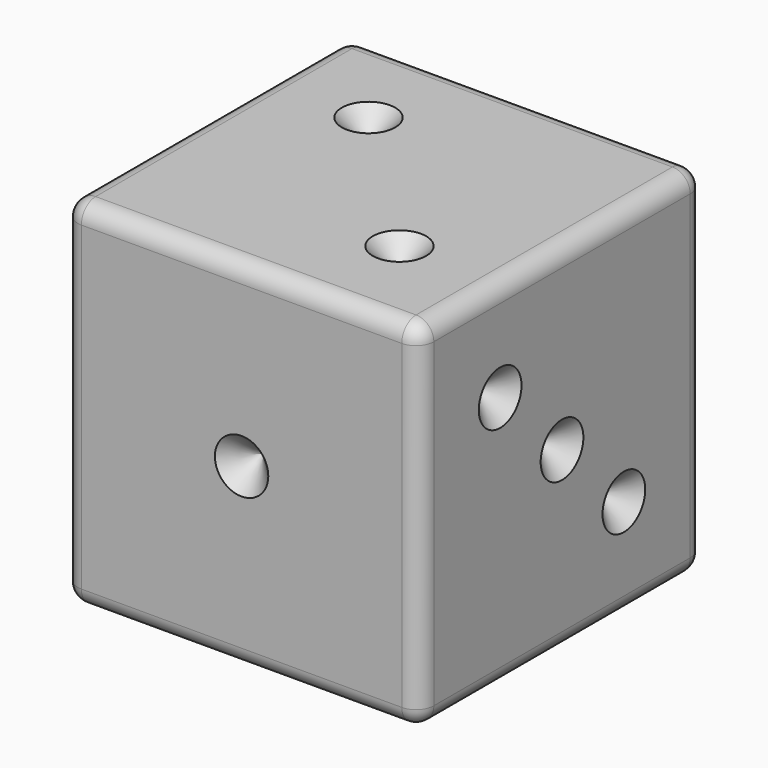
from build123d import *

# Parameters (mm, degrees)
F0_W      = 20
F0_H      = 20
F1_DEPTH  = 20
F2_R      = 1.5
F3_DEPTH  = 1.5
F4_R      = 1
F5_R      = 1.5
F6_DEPTH  = 1.5
F7_R      = 1.5
F8_DEPTH  = 1.5
F9_R      = 1.5
F10_DEPTH = 1.5
F11_R     = 1.5
F12_DEPTH = 1.5
F13_R     = 1.5
F14_DEPTH = 1.5
F15_SIZE  = 1.49999


# Not quite as in the source:
# - a fillet or chamfer is up to 0.001 mm smaller than in the source, because OpenCascade refuses the exact size


with BuildPart() as f1:
    # F0 (on Top) → F1 (new body)
    with BuildSketch(Plane.XY):
        with Locations((10, 10)):
            Rectangle(F0_W, F0_H)
    extrude(amount=F1_DEPTH)

    # F2 (on face) → F3 (cut)
    with BuildSketch(Plane.XZ):
        with Locations((10, 10)):
            Circle(F2_R)
    extrude(amount=-F3_DEPTH, mode=Mode.SUBTRACT)

    # F4
    f4_edges = [f1.edges().sort_by_distance(p)[0] for p in [
        (10, 0, 20),
        (20, 10, 20),
        (20, 0, 10),
        (0, 0, 10),
        (10, 0, 0),
        (20, 10, 0),
        (0, 10, 20),
        (10, 20, 20),
        (0, 10, 0),
        (0, 20, 10),
        (20, 20, 10),
        (10, 20, 0),
    ]]
    fillet(f4_edges, radius=F4_R)

    # F5 (on face) → F6 (cut)
    with BuildSketch(Plane.XY.offset(20)):
        with Locations((5.6568542495, 14.3431457505)):
            Circle(F5_R)
        with Locations((14.3431457505, 5.6568542495)):
            Circle(F5_R)
    extrude(amount=-F6_DEPTH, mode=Mode.SUBTRACT)

    # F7 (on face) → F8 (cut)
    with BuildSketch(Plane.YZ.offset(20)):
        with Locations((5.6568542495, 14.3431457505)):
            Circle(F7_R)
        with Locations((10, 10)):
            Circle(F7_R)
        with Locations((14.3431457505, 5.6568542495)):
            Circle(F7_R)
    extrude(amount=-F8_DEPTH, mode=Mode.SUBTRACT)

    # F9 (on face) → F10 (cut)
    with BuildSketch(Plane(origin=(0, 0, 0), x_dir=(0, -1, 0), z_dir=(-1, 0, 0))):
        with Locations((-14.3431457505, 14.3431457505)):
            Circle(F9_R)
        with Locations((-5.6568542495, 14.3431457505)):
            Circle(F9_R)
        with Locations((-14.3431457505, 5.6568542495)):
            Circle(F9_R)
        with Locations((-5.6568542495, 5.6568542495)):
            Circle(F9_R)
    extrude(amount=-F10_DEPTH, mode=Mode.SUBTRACT)

    # F11 (on face) → F12 (cut)
    with BuildSketch(Plane(origin=(0, 0, 0), x_dir=(1, 0, 0), z_dir=(0, 0, -1))):
        with Locations((5.6568542495, -5.6568542495)):
            Circle(F11_R)
        with Locations((10, -10)):
            Circle(F11_R)
        with Locations((14.3431457505, -5.6568542495)):
            Circle(F11_R)
        with Locations((5.6568542495, -14.3431457505)):
            Circle(F11_R)
        with Locations((14.3431457505, -14.3431457505)):
            Circle(F11_R)
    extrude(amount=-F12_DEPTH, mode=Mode.SUBTRACT)

    # F13 (on face) → F14 (cut)
    with BuildSketch(Plane(origin=(0, 20, 0), x_dir=(-1, 0, 0), z_dir=(0, 1, 0))):
        with Locations((-5.6367907673, 14.3558382988)):
            Circle(F13_R)
        with Locations((-10, 14.3431457505)):
            Circle(F13_R)
        with Locations((-14.1635667533, 14.496743679)):
            Circle(F13_R)
        with Locations((-14.3617270514, 5.7898699306)):
            Circle(F13_R)
        with Locations((-9.9599251616, 5.6883007245)):
            Circle(F13_R)
        with Locations((-5.8349510655, 5.6489654817)):
            Circle(F13_R)
    extrude(amount=-F14_DEPTH, mode=Mode.SUBTRACT)

    # F15 (size 1.5 in the source; OpenCascade refuses exactly that, so slightly less here)
    f15_edges = [f1.edges().sort_by_distance(p)[0] for p in [
        (8.5, 1.5, 10),
        (4.156854, 14.343146, 18.5),
        (12.843146, 5.656854, 18.5),
        (18.5, 4.156854, 14.343146),
        (18.5, 8.5, 10),
        (18.5, 12.843146, 5.656854),
        (1.5, 15.843146, 5.656854),
        (1.5, 15.843146, 14.343146),
        (1.5, 7.156854, 14.343146),
        (1.5, 7.156854, 5.656854),
        (4.156854, 5.656854, 1.5),
        (12.843146, 5.656854, 1.5),
        (8.5, 10, 1.5),
        (4.156854, 14.343146, 1.5),
        (12.843146, 14.343146, 1.5),
        (7.136791, 18.5, 14.355838),
        (11.5, 18.5, 14.343146),
        (15.663567, 18.5, 14.496744),
        (15.861727, 18.5, 5.78987),
        (11.459925, 18.5, 5.688301),
        (7.334951, 18.5, 5.648965),
    ]]
    chamfer(f15_edges, length=F15_SIZE)


solid = f1.part
